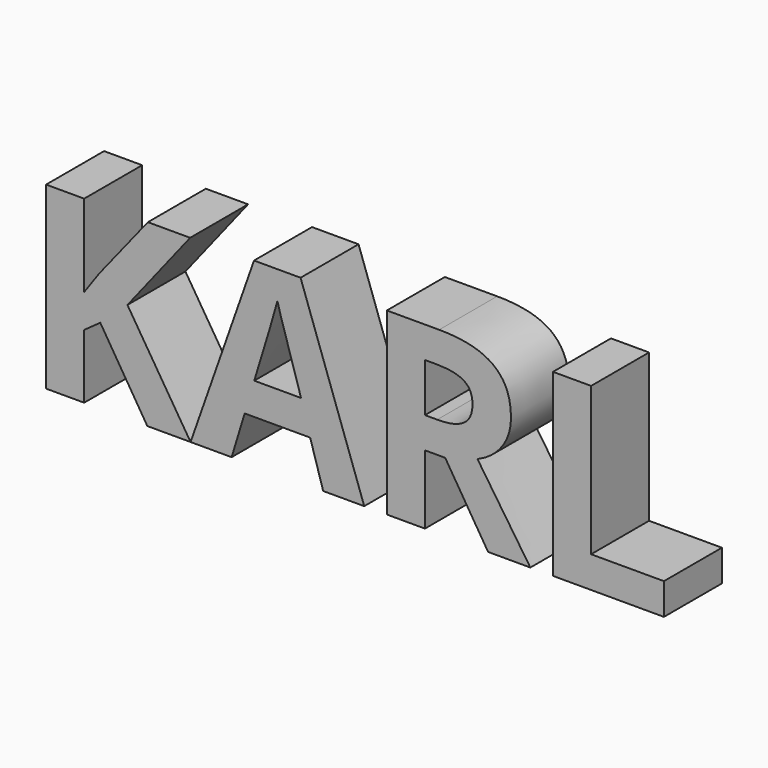
from build123d import *

# Parameters (mm, degrees)
F0_TEXT_SIZE = 34.7222222222
F1_DEPTH     = 10


# Not quite as in the source:
# - Text() gives the source's letters only with a copy of the font that has no kerning and outlines rounded to 1/6400 em; it was checked with that copy


with BuildPart() as f1:
    # F0 (on Front) → F1 (new body)
    with BuildSketch(Plane.XZ):
        with Locations((-71.3365173656, 0)):
            Text('KARL', F0_TEXT_SIZE, font='Open Sans', font_style=FontStyle.BOLD, text_align=(TextAlign.LEFT, TextAlign.BOTTOM))
    extrude(amount=F1_DEPTH)


solid = f1.part
